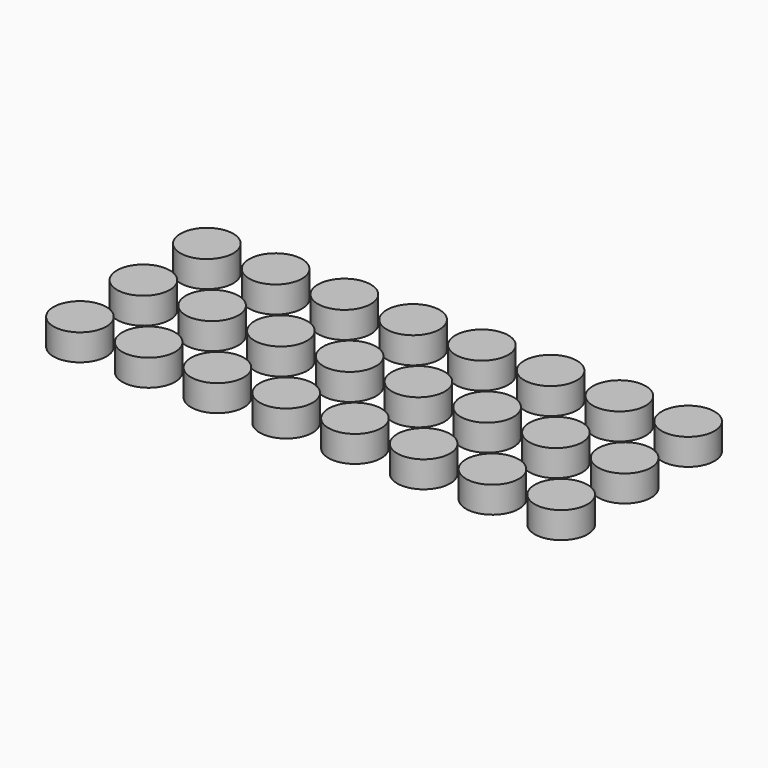
from build123d import *

# Parameters (mm, degrees)
F0_R     = 12.7
F1_DEPTH = 12.7


# Not quite as in the source:
# - a feature names something its author has since deleted; it is built from what else it names


with BuildPart() as f1:
    # F0 (on Top) → F1 (new body)
    with BuildSketch(Plane.XY):
        with Locations((231.14, 0)):
            Circle(F0_R)
    extrude(amount=F1_DEPTH)


with BuildPart() as f1b:
    # F0 (on Top) → F1, piece 2 (new body)
    with BuildSketch(Plane.XY):
        with Locations((198.12, 0)):
            Circle(F0_R)
    extrude(amount=F1_DEPTH)


with BuildPart() as f1c:
    # F0 (on Top) → F1, piece 3 (new body)
    with BuildSketch(Plane.XY):
        with Locations((165.1, 0)):
            Circle(F0_R)
    extrude(amount=F1_DEPTH)


with BuildPart() as f1d:
    # F0 (on Top) → F1, piece 4 (new body)
    with BuildSketch(Plane.XY):
        with Locations((132.08, 0)):
            Circle(F0_R)
    extrude(amount=F1_DEPTH)


with BuildPart() as f1e:
    # F0 (on Top) → F1, piece 5 (new body)
    with BuildSketch(Plane.XY):
        with Locations((99.06, 0)):
            Circle(F0_R)
    extrude(amount=F1_DEPTH)


with BuildPart() as f1f:
    # F0 (on Top) → F1, piece 6 (new body)
    with BuildSketch(Plane.XY):
        with Locations((33.02, 0)):
            Circle(F0_R)
    extrude(amount=F1_DEPTH)


with BuildPart() as f1g:
    # F0 (on Top) → F1, piece 7 (new body)
    with BuildSketch(Plane.XY):
        with Locations((66.04, 0)):
            Circle(F0_R)
    extrude(amount=F1_DEPTH)


with BuildPart() as f1h:
    # F0 (on Top) → F1, piece 8 (new body)
    with BuildSketch(Plane.XY):
        Circle(F0_R)
    extrude(amount=F1_DEPTH)


with BuildPart() as f1i:
    # F0 (on Top) → F1, piece 9 (new body)
    with BuildSketch(Plane.XY):
        with Locations((0, 38.1)):
            Circle(F0_R)
    extrude(amount=F1_DEPTH)


with BuildPart() as f1j:
    # F0 (on Top) → F1, piece 10 (new body)
    with BuildSketch(Plane.XY):
        with Locations((33.02, 38.1)):
            Circle(F0_R)
    extrude(amount=F1_DEPTH)


with BuildPart() as f1k:
    # F0 (on Top) → F1, piece 11 (new body)
    with BuildSketch(Plane.XY):
        with Locations((66.04, 38.1)):
            Circle(F0_R)
    extrude(amount=F1_DEPTH)


with BuildPart() as f1l:
    # F0 (on Top) → F1, piece 12 (new body)
    with BuildSketch(Plane.XY):
        with Locations((99.06, 38.1)):
            Circle(F0_R)
    extrude(amount=F1_DEPTH)


with BuildPart() as f1m:
    # F0 (on Top) → F1, piece 13 (new body)
    with BuildSketch(Plane.XY):
        with Locations((132.08, 38.1)):
            Circle(F0_R)
    extrude(amount=F1_DEPTH)


with BuildPart() as f1n:
    # F0 (on Top) → F1, piece 14 (new body)
    with BuildSketch(Plane.XY):
        with Locations((165.1, 38.1)):
            Circle(F0_R)
    extrude(amount=F1_DEPTH)


with BuildPart() as f1o:
    # F0 (on Top) → F1, piece 15 (new body)
    with BuildSketch(Plane.XY):
        with Locations((198.12, 38.1)):
            Circle(F0_R)
    extrude(amount=F1_DEPTH)


with BuildPart() as f1p:
    # F0 (on Top) → F1, piece 16 (new body)
    with BuildSketch(Plane.XY):
        with Locations((231.14, 38.1)):
            Circle(F0_R)
    extrude(amount=F1_DEPTH)


with BuildPart() as f1q:
    # F0 (on Top) → F1, piece 17 (new body)
    with BuildSketch(Plane.XY):
        with Locations((198.12, 76.2)):
            Circle(F0_R)
    extrude(amount=F1_DEPTH)


with BuildPart() as f1r:
    # F0 (on Top) → F1, piece 18 (new body)
    with BuildSketch(Plane.XY):
        with Locations((165.1, 76.2)):
            Circle(F0_R)
    extrude(amount=F1_DEPTH)


with BuildPart() as f1s:
    # F0 (on Top) → F1, piece 19 (new body)
    with BuildSketch(Plane.XY):
        with Locations((132.08, 76.2)):
            Circle(F0_R)
    extrude(amount=F1_DEPTH)


with BuildPart() as f1t:
    # F0 (on Top) → F1, piece 20 (new body)
    with BuildSketch(Plane.XY):
        with Locations((99.06, 76.2)):
            Circle(F0_R)
    extrude(amount=F1_DEPTH)


with BuildPart() as f1u:
    # F0 (on Top) → F1, piece 21 (new body)
    with BuildSketch(Plane.XY):
        with Locations((66.04, 76.2)):
            Circle(F0_R)
    extrude(amount=F1_DEPTH)


with BuildPart() as f1v:
    # F0 (on Top) → F1, piece 22 (new body)
    with BuildSketch(Plane.XY):
        with Locations((33.02, 76.2)):
            Circle(F0_R)
    extrude(amount=F1_DEPTH)


with BuildPart() as f1w:
    # F0 (on Top) → F1, piece 23 (new body)
    with BuildSketch(Plane.XY):
        with Locations((0, 76.2)):
            Circle(F0_R)
    extrude(amount=F1_DEPTH)


with BuildPart() as f1x:
    # F0 (on Top) → F1, piece 24 (new body)
    with BuildSketch(Plane.XY):
        with Locations((231.14, 76.2)):
            Circle(F0_R)
    extrude(amount=F1_DEPTH)


solid = Compound([f1.part, f1b.part, f1c.part, f1d.part, f1e.part, f1f.part, f1g.part, f1h.part, f1i.part, f1j.part, f1k.part, f1l.part, f1m.part, f1n.part, f1o.part, f1p.part, f1q.part, f1r.part, f1s.part, f1t.part, f1u.part, f1v.part, f1w.part, f1x.part])
